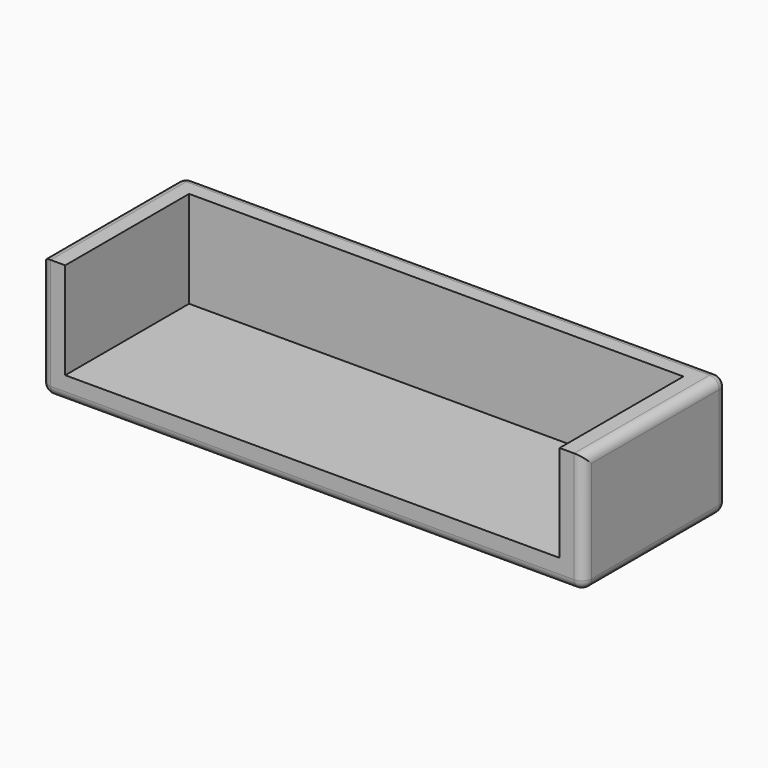
from build123d import *

# Parameters (mm, degrees)
F0_W         = 102.2
F0_H         = 32
F1_DEPTH     = 5
F2_W         = 32
F2_H         = 25
F3_DEPTH     = 5
F4_W         = 32
F4_H         = 25
F5_DEPTH     = 5
F6_W         = 112.2
F6_H         = 25
F7_DEPTH     = 5
F8_R         = 2
F9_TEXT_SIZE = 22.3599154399
F10_DEPTH    = 2.5


# Not quite as in the source:
# - Text() gives the source's letters only with a copy of the font that has no kerning and outlines rounded to 1/6400 em; it was checked with that copy


with BuildPart() as f1:
    # F0 (on Top) → F1 (new body)
    with BuildSketch(Plane.XY):
        with Locations((24.2969034593, 12.9738678224)):
            Rectangle(F0_W, F0_H)
    extrude(amount=F1_DEPTH)

    # F2 (on face) → F3 (join)
    with BuildSketch(Plane.YZ.offset(75.3969034593)):
        with Locations((12.9738678224, 12.5)):
            Rectangle(F2_W, F2_H)
    extrude(amount=F3_DEPTH)

    # F4 (on face) → F5 (join)
    with BuildSketch(Plane(origin=(-26.8030965407, 0, 0), x_dir=(0, -1, 0), z_dir=(-1, 0, 0))):
        with Locations((-12.9738678224, 12.5)):
            Rectangle(F4_W, F4_H)
    extrude(amount=F5_DEPTH)

    # F6 (on face) → F7 (join)
    with BuildSketch(Plane(origin=(0, 28.9738678224, 0), x_dir=(-1, 0, 0), z_dir=(0, 1, 0))):
        with Locations((-24.2969034593, 12.5)):
            Rectangle(F6_W, F6_H)
    extrude(amount=F7_DEPTH)

    # F8
    f8_edges = [f1.edges().sort_by_distance(p)[0] for p in [
        (-31.803097, 15.473868, 25),
        (80.396903, 15.473868, 25),
        (24.296903, 33.973868, 25),
        (24.296903, -3.026132, 0),
        (-31.803097, 15.473868, 0),
        (-31.803097, -3.026132, 12.5),
        (80.396903, 15.473868, 0),
        (24.296903, 33.973868, 0),
        (80.396903, 33.973868, 12.5),
        (-31.803097, 33.973868, 12.5),
        (80.396903, -3.026132, 12.5),
    ]]
    fillet(f8_edges, radius=F8_R)

    # F9 (on face) → F10 (cut)
    with BuildSketch(Plane(origin=(0, 0, 0), x_dir=(1, 0, 0), z_dir=(0, 0, -1))):
        with Locations((-22.2276616842, -23.7607769668)):
            Text('WESLEY', F9_TEXT_SIZE, font='Tinos', font_style=FontStyle.BOLDITALIC, text_align=(TextAlign.LEFT, TextAlign.BOTTOM))
    extrude(amount=-F10_DEPTH, mode=Mode.SUBTRACT)


solid = f1.part
